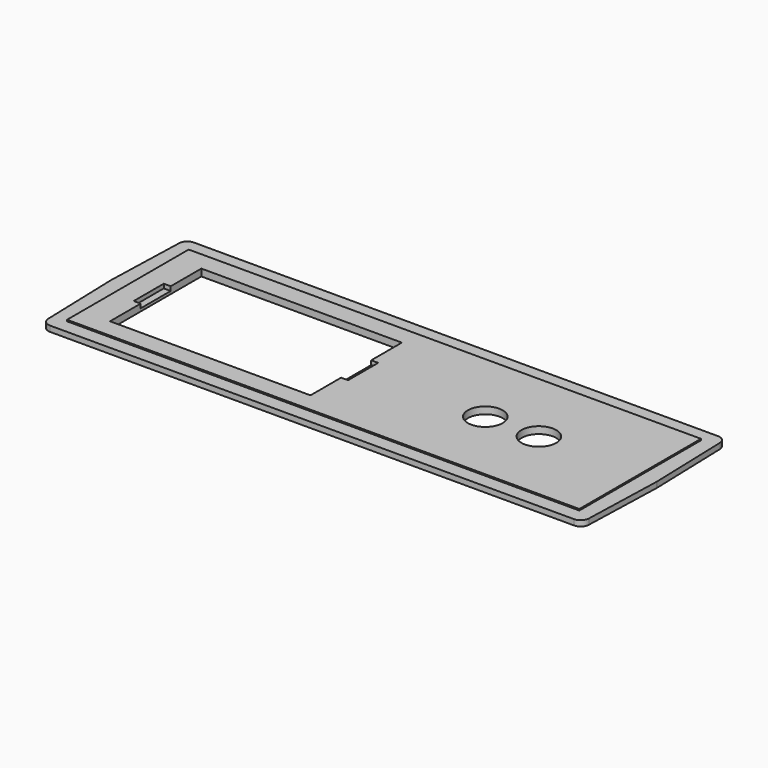
from build123d import *

# Parameters (mm, degrees)
F0_W        = 194
F0_H        = 64.6
F1_DEPTH    = 2
F2_W        = 184
F2_H        = 54.6
F3_DEPTH    = 0.5
F4_R        = 6.25
F4_W        = 2.5
F4_H        = 13.5
F5_DEPTH    = 25
F6_T1_DEPTH = 16.5427907903
F6_T3_DEPTH = 2.4643962848
F7_DEPTH    = 1.5


# Not quite as in the source:
# - a fillet or chamfer that OpenCascade refuses, or shapes differently, is made with other operations: its cross-section is extruded or revolved along the edge and cut away or added


with BuildPart() as f1:
    # F0 (on Top) → F1 (new body)
    with BuildSketch(Plane.XY):
        Rectangle(F0_W, F0_H)
        Polygon((98, 0), (97, 32.3), (97, -32.3), align=None)
        Polygon((-97, -32.3), (-97, 32.3), (-98, 0), align=None)
    extrude(amount=F1_DEPTH)

    # F2 (on face) → F3 (join)
    with BuildSketch(Plane.XY.offset(2)):
        Rectangle(F2_W, F2_H)
    extrude(amount=F3_DEPTH)

    # F4 (on face) → F5 (cut)
    with BuildSketch(Plane.XY.offset(2.5)):
        Polygon((-10, 20.5), (-82, 20.5), (-82, 6.75), (-79.5, 6.75), (-79.5, -6.75), (-82, -6.75), (-82, -20.5), (-10, -20.5), (-10, -6.75), (-12.5, -6.75), (-12.5, 6.75), (-10, 6.75), align=None)
        with Locations((36.375, 0)):
            Circle(F4_R)
        with Locations((55.625, 0)):
            Circle(F4_R)
        with Locations((-11.25, 0)):
            Rectangle(F4_W, F4_H)
        with Locations((-80.75, 0)):
            Rectangle(F4_W, F4_H)
    extrude(amount=-F5_DEPTH, mode=Mode.SUBTRACT)

    # F6: fillet of radius 3 on 6 edges, made by hand

    # F6_s2 → F6_t1 (cut)
    with BuildSketch(Plane.XY.offset(-7.2713953952)):
        with BuildLine():
            ThreePointArc((97.0900051153, -29.3928347763), (96.1796822102, -31.4538923289), (94.0914418419, -32.3))
            Line((94.0914418419, -32.3), (97, -32.3))
            Line((97, -32.3), (97.0900051153, -29.3928347763))
        make_face()
        with BuildLine():
            ThreePointArc((94.0914418419, 32.3), (96.1796822102, 31.4538923289), (97.0900051153, 29.3928347763))
            Line((97.0900051153, 29.3928347763), (97, 32.3))
            Line((97, 32.3), (94.0914418419, 32.3))
        make_face()
        with BuildLine():
            ThreePointArc((-94.0914418419, 32.3), (-96.1796822102, 31.4538923289), (-97.0900051153, 29.3928347763))
            Line((-97.0900051153, 29.3928347763), (-97, 32.3))
            Line((-97, 32.3), (-94.0914418419, 32.3))
        make_face()
        with BuildLine():
            ThreePointArc((-97.0900051153, -29.3928347763), (-96.1796822102, -31.4538923289), (-94.0914418419, -32.3))
            Line((-94.0914418419, -32.3), (-97, -32.3))
            Line((-97, -32.3), (-97.0900051153, -29.3928347763))
        make_face()
    extrude(amount=F6_T1_DEPTH, mode=Mode.SUBTRACT)

    # F6_s4 → F6_t3 (cut)
    with BuildSketch(Plane.XY.offset(-0.2321981424)):
        with BuildLine():
            ThreePointArc((-97.9971258583, 0.0928347763), (-97.998562585, 0), (-97.9971258583, -0.0928347763))
            Line((-97.9971258583, -0.0928347763), (-98, 0))
            Line((-98, 0), (-97.9971258583, 0.0928347763))
        make_face()
        with BuildLine():
            ThreePointArc((97.9971258583, 0.0928347763), (97.998562585, 0), (97.9971258583, -0.0928347763))
            Line((97.9971258583, -0.0928347763), (98, 0))
            Line((98, 0), (97.9971258583, 0.0928347763))
        make_face()
    extrude(amount=F6_T3_DEPTH, mode=Mode.SUBTRACT)

    # F4 (on face) → F7 (cut)
    with BuildSketch(Plane.XY.offset(2.5)):
        Polygon((-10, 20.5), (-82, 20.5), (-82, 6.75), (-79.5, 6.75), (-79.5, -6.75), (-82, -6.75), (-82, -20.5), (-10, -20.5), (-10, -6.75), (-12.5, -6.75), (-12.5, 6.75), (-10, 6.75), align=None)
        with Locations((-80.75, 0)):
            Rectangle(F4_W, F4_H)
        with Locations((-83.25, 0)):
            Rectangle(F4_W, F4_H)
        with Locations((-8.75, 0)):
            Rectangle(F4_W, F4_H)
        with Locations((-11.25, 0)):
            Rectangle(F4_W, F4_H)
        with Locations((36.375, 0)):
            Circle(F4_R)
        with Locations((55.625, 0)):
            Circle(F4_R)
    extrude(amount=-F7_DEPTH, mode=Mode.SUBTRACT)


solid = f1.part
